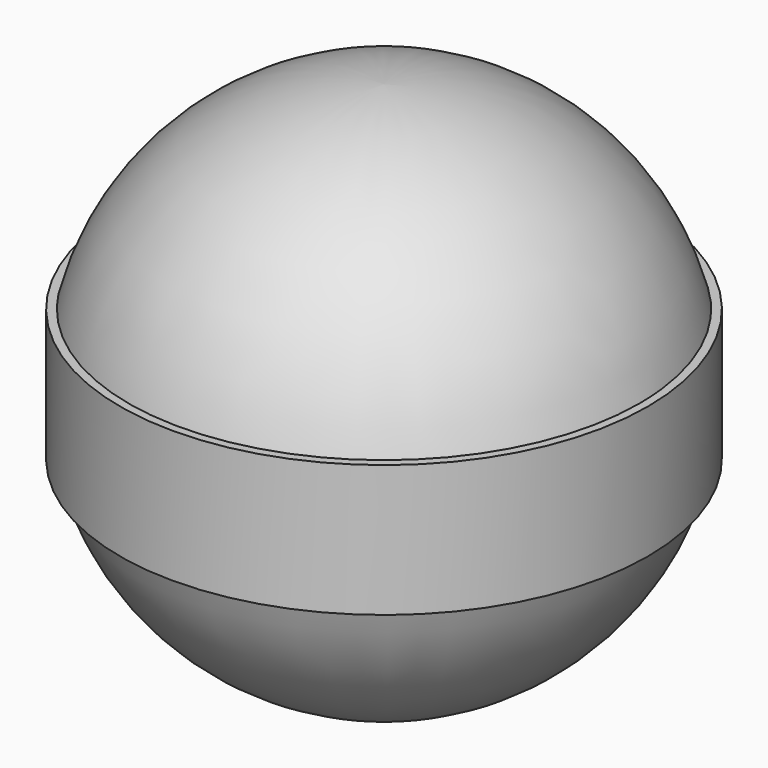
from build123d import *

# Parameters (mm, degrees)
F0_R     = 6.35
F1_DEPTH = 6.35
F2_R     = 6.34999
F3_R     = 6.35
F4_DEPTH = 1.5875


# Not quite as in the source:
# - a fillet or chamfer is up to 0.001 mm smaller than in the source, because OpenCascade refuses the exact size


with BuildPart() as f1:
    # F0 (on Top) → F1 (new body, symmetric)
    with BuildSketch(Plane.XY):
        Circle(F0_R)
    extrude(amount=F1_DEPTH, both=True)

    # F2 (radius 6.35 in the source; OpenCascade refuses exactly that, so slightly less here)
    f2_edges = [f1.edges().sort_by_distance(p)[0] for p in [
        (-6.35, 0, 6.35),
        (-6.35, 0, -6.35),
    ]]
    fillet(f2_edges, radius=F2_R)

    # F3 (on Top) → F4 (join, symmetric)
    with BuildSketch(Plane.XY):
        Circle(F3_R)
    extrude(amount=F4_DEPTH, both=True)


solid = f1.part
